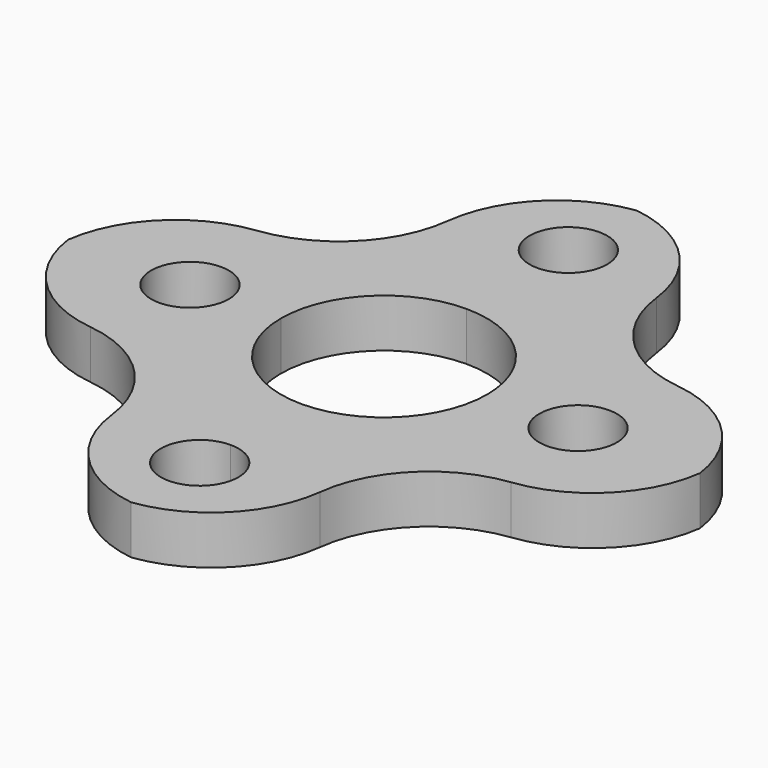
from build123d import *

# Parameters (mm, degrees)
F1_R        = 13.1
F1_R_2      = 1.6
F2_DEPTH    = 2
F3_R        = 5
F4_DEPTH    = 25
F5_T1_DEPTH = 33.3713058975


# Not quite as in the source:
# - a fillet or chamfer that OpenCascade refuses, or shapes differently, is made with other operations: its cross-section is extruded or revolved along the edge and cut away or added


with BuildPart() as f2:
    # F1 (on Top) → F2 (new body)
    with BuildSketch(Plane.XY):
        Circle(F1_R)
        with BuildLine():
            ThreePointArc((1.6, -9.5), (-1.1313708499, -10.6313708499), (0, -7.9))
            ThreePointArc((0, -7.9), (1.1313708499, -8.3686291501), (1.6, -9.5))
        make_face(mode=Mode.SUBTRACT)
        with Locations((-8, 0)):
            Circle(F1_R_2, mode=Mode.SUBTRACT)
        with BuildLine():
            ThreePointArc((-4.25, 0), (-3.00520382, 3.00520382), (0, 4.25))
            ThreePointArc((0, 4.25), (3.00520382, 3.00520382), (4.25, 0))
            ThreePointArc((4.25, 0), (3.00520382, -3.00520382), (0, -4.25))
            ThreePointArc((0, -4.25), (-3.00520382, -3.00520382), (-4.25, 0))
        make_face(mode=Mode.SUBTRACT)
        with BuildLine():
            ThreePointArc((9.6, 0), (8, -1.6), (6.4, 0))
            ThreePointArc((6.4, 0), (8, 1.6), (9.6, 0))
        make_face(mode=Mode.SUBTRACT)
        with BuildLine():
            ThreePointArc((1.6, 9.5), (1.1313708499, 8.3686291501), (0, 7.9))
            ThreePointArc((0, 7.9), (-1.1313708499, 10.6313708499), (1.6, 9.5))
        make_face(mode=Mode.SUBTRACT)
    extrude(amount=F2_DEPTH)

    # F3 (on face) → F4 (cut)
    with BuildSketch(Plane.XY.offset(2)):
        with Locations((-9.2630988335, 9.2630988335)):
            Circle(F3_R)
        with Locations((9.2630988335, -9.2630988335)):
            Circle(F3_R)
        with Locations((-9.2630988335, -9.2630988335)):
            Circle(F3_R)
        with Locations((9.2630988335, 9.2630988335)):
            Circle(F3_R)
    extrude(amount=-F4_DEPTH, mode=Mode.SUBTRACT)

    # F5: fillet of radius 5 on 8 edges, made by hand

    # F5_s2 → F5_t1 (cut)
    with BuildSketch(Plane.XY.offset(-15.6856529487)):
        with BuildLine():
            ThreePointArc((1.0767599787, 13.0556726348), (-2.4959833234, 11.9459923629), (-4.298657973, 8.667845155))
            ThreePointArc((-4.298657973, 8.667845155), (-4.4028928152, 10.437150561), (-5.1178235319, 12.0589337131))
            ThreePointArc((-5.1178235319, 12.0589337131), (-2.0810864422, 12.9336413751), (1.0767599787, 13.0556726348))
        make_face()
        with BuildLine():
            ThreePointArc((-8.667845155, 4.298657973), (-11.9459923629, 2.4959833234), (-13.0556726348, -1.0767599787))
            ThreePointArc((-13.0556726348, -1.0767599787), (-12.9336413751, 2.0810864422), (-12.0589337131, 5.1178235319))
            ThreePointArc((-12.0589337131, 5.1178235319), (-10.437150561, 4.4028928152), (-8.667845155, 4.298657973))
        make_face()
        with BuildLine():
            ThreePointArc((13.0556726348, -1.0767599787), (11.9459923629, 2.4959833234), (8.667845155, 4.298657973))
            ThreePointArc((8.667845155, 4.298657973), (10.437150561, 4.4028928152), (12.0589337131, 5.1178235319))
            ThreePointArc((12.0589337131, 5.1178235319), (12.9336413751, 2.0810864422), (13.0556726348, -1.0767599787))
        make_face()
        with BuildLine():
            ThreePointArc((4.298657973, 8.667845155), (2.4959833234, 11.9459923629), (-1.0767599787, 13.0556726348))
            ThreePointArc((-1.0767599787, 13.0556726348), (2.0810864422, 12.9336413751), (5.1178235319, 12.0589337131))
            ThreePointArc((5.1178235319, 12.0589337131), (4.4028928152, 10.437150561), (4.298657973, 8.667845155))
        make_face()
        with BuildLine():
            ThreePointArc((13.0556726348, 1.0767599787), (11.9459923629, -2.4959833234), (8.667845155, -4.298657973))
            ThreePointArc((8.667845155, -4.298657973), (10.437150561, -4.4028928152), (12.0589337131, -5.1178235319))
            ThreePointArc((12.0589337131, -5.1178235319), (12.9336413751, -2.0810864422), (13.0556726348, 1.0767599787))
        make_face()
        with BuildLine():
            ThreePointArc((-1.0767599787, -13.0556726348), (2.4959833234, -11.9459923629), (4.298657973, -8.667845155))
            ThreePointArc((4.298657973, -8.667845155), (4.4028928152, -10.437150561), (5.1178235319, -12.0589337131))
            ThreePointArc((5.1178235319, -12.0589337131), (2.0810864422, -12.9336413751), (-1.0767599787, -13.0556726348))
        make_face()
        with BuildLine():
            ThreePointArc((-13.0556726348, 1.0767599787), (-11.9459923629, -2.4959833234), (-8.667845155, -4.298657973))
            ThreePointArc((-8.667845155, -4.298657973), (-10.437150561, -4.4028928152), (-12.0589337131, -5.1178235319))
            ThreePointArc((-12.0589337131, -5.1178235319), (-12.9336413751, -2.0810864422), (-13.0556726348, 1.0767599787))
        make_face()
        with BuildLine():
            ThreePointArc((-4.298657973, -8.667845155), (-2.4959833234, -11.9459923629), (1.0767599787, -13.0556726348))
            ThreePointArc((1.0767599787, -13.0556726348), (-2.0810864422, -12.9336413751), (-5.1178235319, -12.0589337131))
            ThreePointArc((-5.1178235319, -12.0589337131), (-4.4028928152, -10.437150561), (-4.298657973, -8.667845155))
        make_face()
    extrude(amount=F5_T1_DEPTH, mode=Mode.SUBTRACT)


solid = f2.part
